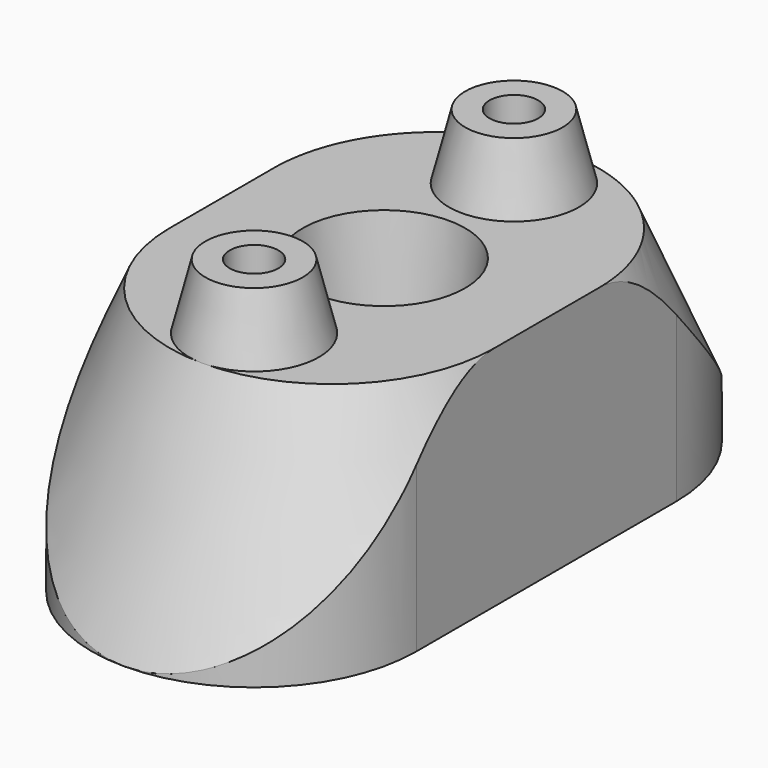
from build123d import *

# Parameters (mm, degrees)
F1_DEPTH      = 44.45
F4_ANGLE_BACK = 90
F4_ANGLE      = 180
F10_D         = 9.525


# Not quite as in the source:
# - a pattern or mirror of a feature is missing from the dataset's text; its kind, count and spacing are read off the source's solid


with BuildPart() as f1:
    # F0 (on Top) → F1 (new body)
    with BuildSketch(Plane.XY):
        with BuildLine():
            Line((-31.75, 63.5), (-31.75, 0))
            ThreePointArc((-31.75, 0), (0, -31.75), (31.75, 0))
            Line((31.75, 0), (31.75, 63.5))
            ThreePointArc((31.75, 63.5), (0, 95.25), (-31.75, 63.5))
        make_face()
    extrude(amount=F1_DEPTH)

    # F3 (on Right) → F4 (revolve, cut)
    with BuildSketch(Plane.YZ, mode=Mode.PRIVATE) as f4_sk:
        Polygon((-31.75, 0), (-12.7, 44.45), (-31.75, 44.45), align=None)
    f4 = revolve(f4_sk.sketch.rotate(Axis((0, 19.05, 31.5998233855), (0, 0, 1)), -F4_ANGLE_BACK), axis=Axis((0, 19.05, 31.5998233855), (0, 0, 1)), revolution_arc=F4_ANGLE, mode=Mode.SUBTRACT)

    # F4_copies: F4 across plane
    add(f4.mirror(Plane(origin=(4e-05, 31.750043, -6e-06), x_dir=(1, -1e-06, 0), z_dir=(1e-06, 1, 0))), mode=Mode.SUBTRACT)

    # F5 (on Right) → F6 (revolve)
    with BuildSketch(Plane.YZ):
        Polygon((-9.525, 57.15), (-12.7, 44.45), (0, 44.45), (0, 57.15), align=None)
    f6 = revolve(axis=Axis((0, 0, 50.8), (0, 0, -1)))

    # F6_copies: F6 across plane
    add(f6.mirror(Plane.ZX.offset(31.75)))

    # F7 (on Right) → F8 (revolve, cut)
    with BuildSketch(Plane.YZ):
        Polygon((20.6375, 0), (31.75, 0), (31.75, 44.45), (15.875, 44.45), align=None)
    revolve(axis=Axis((0, 31.75, 22.225), (0, 0, 1)), mode=Mode.SUBTRACT)

    # F10 (through all)
    with Locations(Plane.XY.offset(57.15)):
        with Locations((0, 0), (0, 63.5)):
            Hole(F10_D / 2)


solid = f1.part
